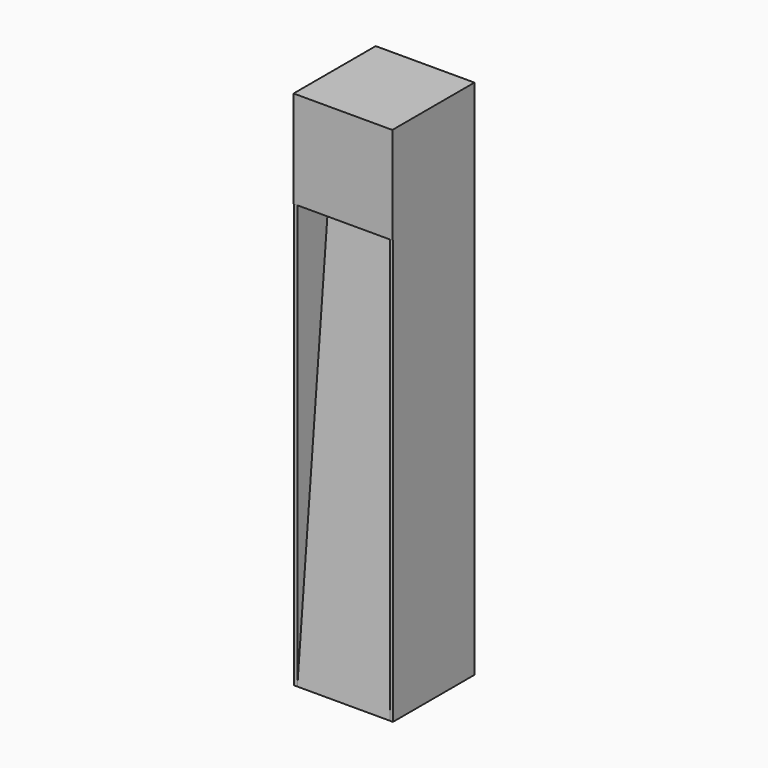
from build123d import *

# Parameters (mm, degrees)
F1_DEPTH = 800
F2_W     = 152.4
F2_H     = 152.4
F3_DEPTH = 4.7625
F4_W     = 152.4
F4_H     = 804.7625
F5_DEPTH = 4.7625
F6_W     = 152.4
F6_H     = 150
F7_DEPTH = 1.21
F9_DEPTH = 71.464


# Not quite as in the source:
# - a length typed as a fraction of an inch, garbled in the dataset ("3 / 203.2 mm" for 3/8 in), is restored


with BuildPart() as f1:
    # F0 (on Top) → F1 (new body)
    with BuildSketch(Plane.XY):
        Polygon((-76.2, 76.2), (-76.2, -76.2), (-71.437, -76.2), (-71.437, -2.3815), (71.437, -2.3815), (71.437, -76.2), (76.2, -76.2), (76.2, 76.2), (71.437, 76.2), (71.437, 2.382), (-71.437, 2.382), (-71.437, 76.2), align=None)
    extrude(amount=-F1_DEPTH)

    # F2 (on face) → F3 (join)
    with BuildSketch(Plane.XY):
        Rectangle(F2_W, F2_H)
    extrude(amount=F3_DEPTH)

    # F4 (on face) → F5 (join)
    with BuildSketch(Plane(origin=(0, 76.2, 0), x_dir=(-1, 0, 0), z_dir=(0, 1, 0))):
        with Locations((0, -397.61875)):
            Rectangle(F4_W, F4_H)
    extrude(amount=F5_DEPTH)

    # F6 (on face) → F7 (join)
    with BuildSketch(Plane.XZ.offset(76.2)):
        with Locations((0, -70.2375)):
            Rectangle(F6_W, F6_H)
    extrude(amount=F7_DEPTH)

    # F8 (on Right) → F9 (join, symmetric)
    with BuildSketch(Plane.YZ):
        Polygon((-76.13632828, -800.0091910362), (-74.92632828, -800.0091910362), (0.8852251628, 4.7220308334), (-0.3247748372, 4.7220308334), align=None)
    extrude(amount=F9_DEPTH, both=True)


solid = f1.part
